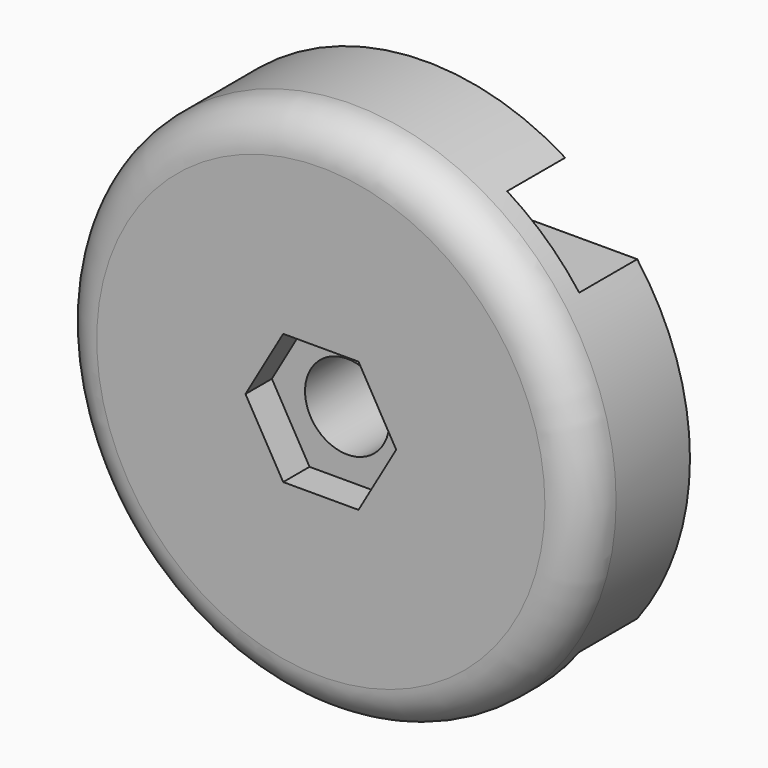
from build123d import *

# Parameters (mm, degrees)
F0_R          = 40
F1_DEPTH      = 20
F2_W          = 11
F2_H          = 10
F3_DEPTH      = 50
F3_DEPTH_BACK = 10
F4_R          = 6
F6_DEPTH      = 5
F7_R          = 6.4
F8_DEPTH      = 25
F9_R          = 1.5
F10_DEPTH     = 16
F11_R         = 3
F12_DEPTH     = 6


# Not quite as in the source:
# - a pattern or mirror of a feature is missing from the dataset's text; its kind, count and spacing are read off the source's solid


with BuildPart() as f1:
    # F0 (on Front) → F1 (new body)
    with BuildSketch(Plane.XZ):
        Circle(F0_R)
    extrude(amount=F1_DEPTH)

    # F2 (on Right) → F3 (cut, two sides)
    with BuildSketch(Plane.YZ) as f3_sk:
        with Locations((-5.5, 29)):
            Rectangle(F2_W, F2_H)
    f3 = extrude(amount=F3_DEPTH, mode=Mode.SUBTRACT) + extrude(f3_sk.sketch, amount=-F3_DEPTH_BACK, mode=Mode.SUBTRACT)

    # F3_copies: F3 across plane
    add(f3.mirror(Plane(origin=(0, 0, 0), x_dir=(-1, 0, 0), z_dir=(0, 0, -1))), mode=Mode.SUBTRACT)

    # F4
    f4_edges = [f1.edges().sort_by_distance(p)[0] for p in [
        (-40, -20, 0),
    ]]
    fillet(f4_edges, radius=F4_R)

    # F5 (on face) → F6 (cut)
    with BuildSketch(Plane.XZ.offset(20)):
        Polygon((-5.715767665, -9.9), (5.715767665, -9.9), (11.43153533, 0), (5.715767665, 9.9), (-5.715767665, 9.9), (-11.43153533, 0), align=None)
    extrude(amount=-F6_DEPTH, mode=Mode.SUBTRACT)

    # F7 (on face) → F8 (cut)
    with BuildSketch(Plane.XZ.offset(15)):
        Circle(F7_R)
    extrude(amount=-F8_DEPTH, mode=Mode.SUBTRACT)

    # F9 (on Front) → F10 (cut)
    with BuildSketch(Plane.XZ):
        with Locations((26, 12)):
            Circle(F9_R)
        with Locations((-26, 12)):
            Circle(F9_R)
        with Locations((-26, -12)):
            Circle(F9_R)
        with Locations((26, -12)):
            Circle(F9_R)
    extrude(amount=F10_DEPTH, mode=Mode.SUBTRACT)

    # F11 (on face) → F12 (cut)
    with BuildSketch(Plane(origin=(0, 0, 0), x_dir=(-1, 0, 0), z_dir=(0, 1, 0))):
        with Locations((-26, 12)):
            Circle(F11_R)
        with Locations((26, 12)):
            Circle(F11_R)
        with Locations((26, -12)):
            Circle(F11_R)
        with Locations((-26, -12)):
            Circle(F11_R)
    extrude(amount=-F12_DEPTH, mode=Mode.SUBTRACT)


solid = f1.part
